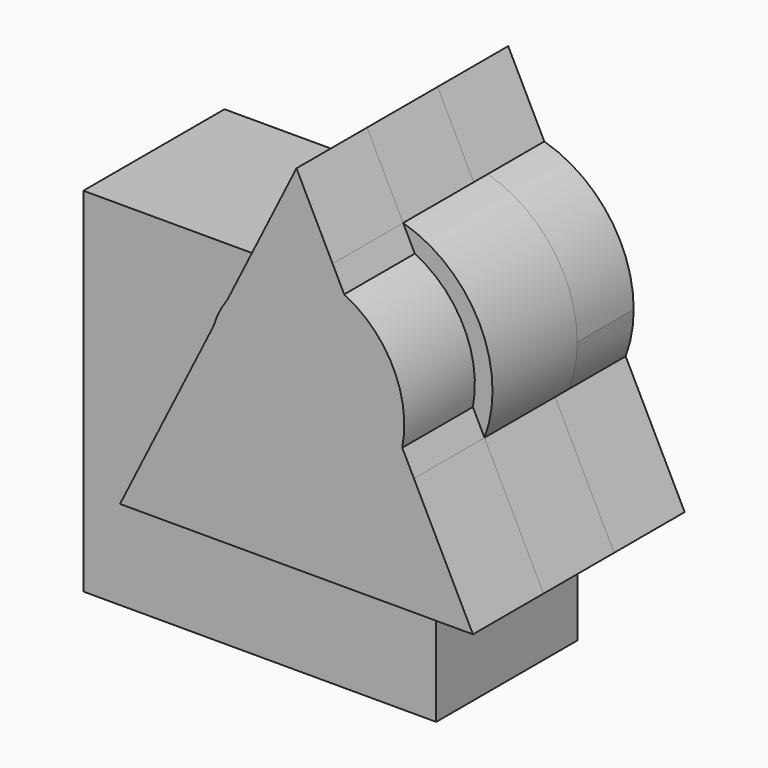
from build123d import *
from build123d import SkipClean  # not in build123d's __all__

# Parameters (mm, degrees)
F1_DEPTH = 50
F2_R     = 10
F3_R     = 20
F4_W     = 200
F4_H     = 200
F5_DEPTH = 100


with BuildPart() as f1:
    # F0 (on Front) → F1 (new body)
    with BuildSketch(Plane.XZ):
        with BuildLine():
            Line((-4.5768408876, 53.0602382816), (-39.2092391849, -16.2045583129))
            Line((-39.2092391849, -16.2045583129), (160.7907608151, -16.2045583129))
            Line((160.7907608151, -16.2045583129), (127.34963023, 50.6777028574))
            ThreePointArc((127.34963023, 50.6777028574), (60.5480822774, 5.4496834996), (-4.5768408876, 53.0602382816))
        make_face()
        with BuildLine():
            ThreePointArc((39.9529426198, 142.1198052965), (-0.8758229979, 106.8719587211), (-4.5768408876, 53.0602382816))
            Line((-4.5768408876, 53.0602382816), (39.9529426198, 142.1198052965))
        make_face()
        with BuildLine():
            Line((39.9529426198, 142.1198052965), (-4.5768408876, 53.0602382816))
            ThreePointArc((-4.5768408876, 53.0602382816), (60.5480822774, 5.4496834996), (127.34963023, 50.6777028574))
            Line((127.34963023, 50.6777028574), (81.2556246585, 142.8657140004))
            ThreePointArc((81.2556246585, 142.8657140004), (60.5480822774, 145.6047584293), (39.9529426198, 142.1198052965))
        make_face()
        with BuildLine():
            Line((81.2556246585, 142.8657140004), (127.34963023, 50.6777028574))
            ThreePointArc((127.34963023, 50.6777028574), (130.7549744187, 62.8956312233), (131.9026168762, 75.5272209644))
            ThreePointArc((131.9026168762, 75.5272209644), (117.8276267442, 117.6567547414), (81.2556246585, 142.8657140004))
        make_face()
        with BuildLine():
            Line((60.7907608151, 183.7954416871), (39.9529426198, 142.1198052965))
            ThreePointArc((39.9529426198, 142.1198052965), (60.5480822774, 145.6047584293), (81.2556246585, 142.8657140004))
            Line((81.2556246585, 142.8657140004), (60.7907608151, 183.7954416871))
        make_face()
    extrude(amount=F1_DEPTH)

    # F2
    f2_edges = [f1.edges().sort_by_distance(p)[0] for p in [
        (124.503128, -50, 106.871959),
    ]]
    fillet(f2_edges, radius=F2_R)

    # F3
    f3_edges = [f1.edges().sort_by_distance(p)[0] for p in [
        (-0.875823, -50, 106.871959),
    ]]
    fillet(f3_edges, radius=F3_R)

    # F4 (on Front) + F1_face (on face) + F1_face1 (on face) → F5 (join)
    with BuildSketch(Plane.XZ):
        Rectangle(F4_W, F4_H)
    with BuildSketch(Plane(origin=(62.2431161931, -50, 51.9688897251), x_dir=(1, 0, 0), z_dir=(0, -1, 0))):
        with BuildLine():
            Line((-22.2901735733, 90.1509155714), (-40.6803150229, 53.3706326721))
            ThreePointArc((-40.6803150229, 53.3706326721), (-45.230395371, 45.958797086), (-48.429815631, 37.8716314558))
            Line((-48.429815631, 37.8716314558), (-66.8199570807, 1.0913485565))
            Line((-66.8199570807, 1.0913485565), (-101.452355378, -68.173448038))
            Line((-101.452355378, -68.173448038), (98.547644622, -68.173448038))
            Line((98.547644622, -68.173448038), (65.1065140369, -1.2911868678))
            Line((65.1065140369, -1.2911868678), (58.5157708494, 11.8902995073))
            ThreePointArc((58.5157708494, 11.8902995073), (53.3157399256, 50.430933041), (25.603251653, 77.7153379001))
            Line((25.603251653, 77.7153379001), (19.0125084654, 90.8968242752))
            Line((19.0125084654, 90.8968242752), (-1.452355378, 131.826551962))
            Line((-1.452355378, 131.826551962), (-22.2901735733, 90.1509155714))
        make_face()
    with BuildSketch(Plane(origin=(61.2741122872, 0, 57.1327908737), x_dir=(1, 0, 0), z_dir=(0, 1, 0))):
        with BuildLine():
            Line((-100.4833514721, 73.3373491866), (-65.8509531748, 4.072552592))
            ThreePointArc((-65.8509531748, 4.072552592), (-62.1499352851, -49.7391678474), (-21.3211696674, -84.9870144228))
            Line((-21.3211696674, -84.9870144228), (-0.4833514721, -126.6626508134))
            Line((-0.4833514721, -126.6626508134), (19.9815123713, -85.7329231267))
            ThreePointArc((19.9815123713, -85.7329231267), (63.2290157415, -49.7391678474), (66.0755179428, 6.4550880163))
            Line((66.0755179428, 6.4550880163), (99.5166485279, 73.3373491866))
            Line((99.5166485279, 73.3373491866), (-100.4833514721, 73.3373491866))
        make_face()
    with SkipClean():  # cleaning this boolean's faces spoils the solid; the shape is the same uncleaned
        extrude(amount=F5_DEPTH, dir=(0, -1, 0))


solid = f1.part
